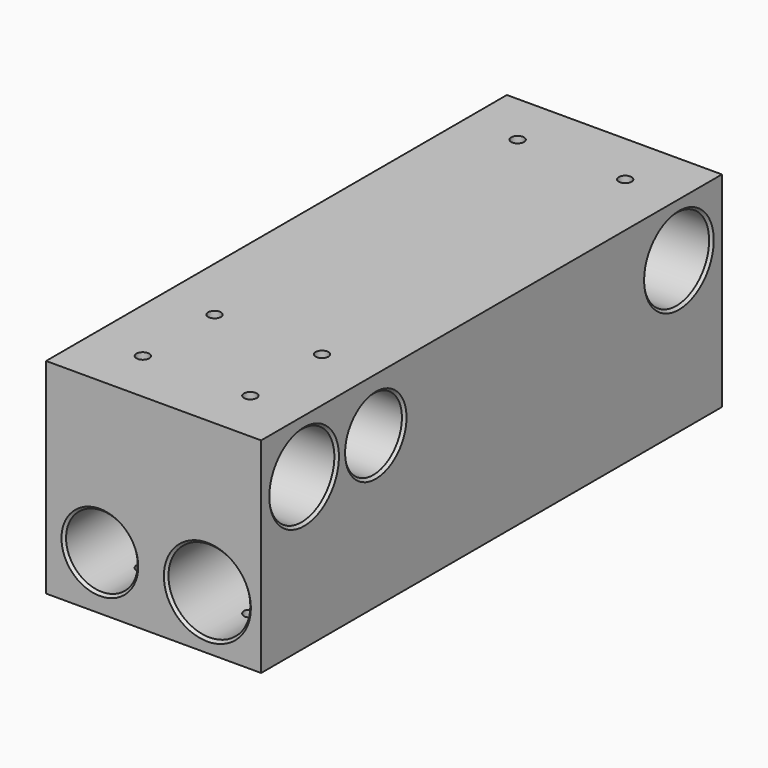
from build123d import *

# Parameters (mm, degrees)
F0_W     = 84
F0_H     = 80
F0_R     = 14
F0_R_2   = 16
F1_DEPTH = 225
F2_R     = 16
F2_R_2   = 14
F3_DEPTH = 100
F4_SIZE  = 1
F5_R     = 2.5
F6_DEPTH = 25
F7_R     = 2.5
F8_DEPTH = 25


# Not quite as in the source:
# - a feature names something its author has since deleted; it is built from what else it names


with BuildPart() as f1:
    # F0 (on Front) → F1 (new body)
    with BuildSketch(Plane.XZ):
        Rectangle(F0_W, F0_H)
        with Locations((-21, -19)):
            Circle(F0_R, mode=Mode.SUBTRACT)
        with Locations((21, -19)):
            Circle(F0_R_2, mode=Mode.SUBTRACT)
    extrude(amount=-F1_DEPTH)

    # F2 (on face) → F3 (cut)
    with BuildSketch(Plane(origin=(-42, 0, 0), x_dir=(0, -1, 0), z_dir=(-1, 0, 0))):
        with Locations((-204, 19)):
            Circle(F2_R)
        with Locations((-56, 19)):
            Circle(F2_R_2)
        with Locations((-21, 19)):
            Circle(F2_R)
    extrude(amount=-F3_DEPTH, mode=Mode.SUBTRACT)

    # F4
    f4_edges = [f1.edges().sort_by_distance(p)[0] for p in [
        (-42, 220, 19),
        (-42, 70, 19),
        (-42, 37, 19),
        (-35, 0, -19),
        (5, 0, -19),
        (42, 37, 19),
        (42, 70, 19),
        (42, 220, 19),
    ]]
    chamfer(f4_edges, length=F4_SIZE)

    # F5 (on face) → F6 (cut)
    with BuildSketch(Plane.XY.offset(40)):
        with Locations((21, 204)):
            Circle(F5_R)
        with Locations((21, 56)):
            Circle(F5_R)
        with Locations((21, 21)):
            Circle(F5_R)
        with Locations((-21, 21)):
            Circle(F5_R)
        with Locations((-21, 56)):
            Circle(F5_R)
        with Locations((-21, 204)):
            Circle(F5_R)
    extrude(amount=-F6_DEPTH, mode=Mode.SUBTRACT)

    # F7 (on face) → F8 (cut)
    with BuildSketch(Plane(origin=(0, 0, -40), x_dir=(1, 0, 0), z_dir=(0, 0, -1))):
        with Locations((-21, -21)):
            Circle(F7_R)
        with Locations((21, -21)):
            Circle(F7_R)
        with BuildLine():
            ThreePointArc((-18.5, -105), (-22.767766953, -103.232233047), (-21, -107.5))
            ThreePointArc((-21, -107.5), (-19.232233047, -106.767766953), (-18.5, -105))
        make_face()
        with BuildLine():
            ThreePointArc((-21, -152.5), (-22.767766953, -156.767766953), (-18.5, -155))
            ThreePointArc((-18.5, -155), (-19.232233047, -153.232233047), (-21, -152.5))
        make_face()
        with Locations((-21, -204)):
            Circle(F7_R)
        with Locations((21, -204)):
            Circle(F7_R)
    extrude(amount=-F8_DEPTH, mode=Mode.SUBTRACT)


solid = f1.part
